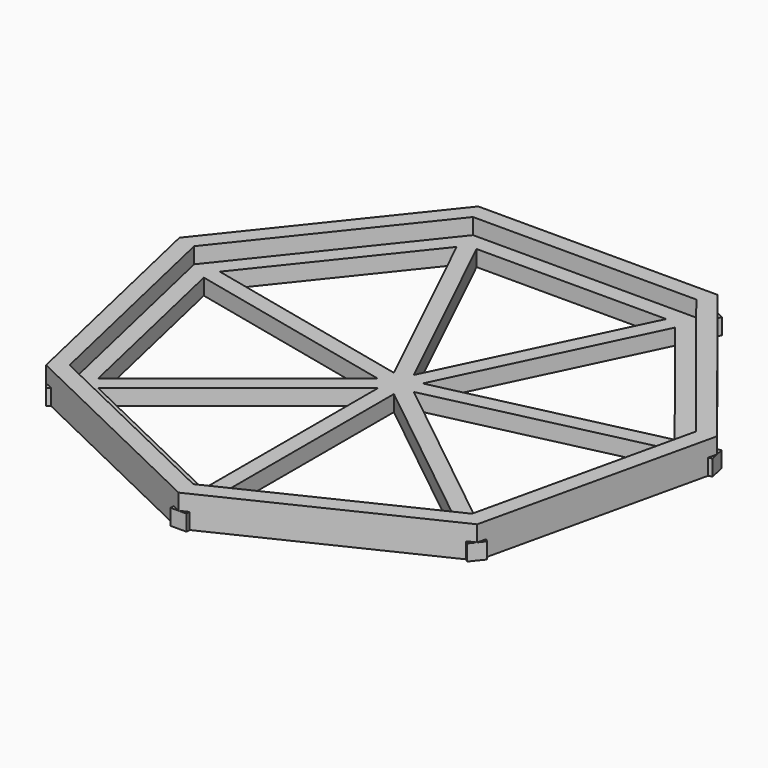
from build123d import *

# Parameters (mm, degrees)
F1_E8_W   = 109.7644269796
F1_E8_H   = 6.35
F2_DEPTH  = 3.175
F1_E7_W   = 109.7644269796
F1_E7_H   = 6.35
F3_DEPTH  = 3.175
F4_E6_W   = 109.7644269796
F4_E6_H   = 6.35
F5_DEPTH  = 3.175
F4_E5_W   = 109.7644269796
F4_E5_H   = 6.35
F6_DEPTH  = 3.175
F7_E4_W   = 109.7644269796
F7_E4_H   = 6.35
F8_DEPTH  = 3.175
F7_E3_W   = 109.7644269796
F7_E3_H   = 6.35
F9_DEPTH  = 3.175
F10_E9_W  = 109.7644269796
F10_E9_H  = 6.35
F11_DEPTH = 3.175
F12_DEPTH = 12.7
F13_DEPTH = 6.35


with BuildPart() as f2:
    # F1_E8 (on explicit) → F2 (new body, symmetric)
    with BuildSketch(Plane(origin=(0, -109.7644269796, 0), x_dir=(0, 1, 0), z_dir=(1, 0, 0))):
        with Locations((54.8822134898, 3.175)):
            Rectangle(F1_E8_W, F1_E8_H)
    extrude(amount=F2_DEPTH, both=True)

    # F1_E7 (on explicit) → F3 (join, symmetric)
    with BuildSketch(Plane(origin=(85.8172846677, -68.4370008286, 0), x_dir=(-0.7818314825, 0.6234898019, 0), z_dir=(0.6234898019, 0.7818314825, 0))):
        with Locations((54.8822134898, 3.175)):
            Rectangle(F1_E7_W, F1_E7_H)
    extrude(amount=F3_DEPTH, both=True)

    # F4_E6 (on explicit) → F5 (join, symmetric)
    with BuildSketch(Plane(origin=(107.012403627, 24.4248828067, 0), x_dir=(-0.9749279122, -0.222520934, 0), z_dir=(-0.222520934, 0.9749279122, 0))):
        with Locations((54.8822134898, 3.175)):
            Rectangle(F4_E6_W, F4_E6_H)
    extrude(amount=F5_DEPTH, both=True)

    # F4_E5 (on explicit) → F6 (join, symmetric)
    with BuildSketch(Plane(origin=(47.625, 98.8943315118, 0), x_dir=(-0.4338837391, -0.9009688679, 0), z_dir=(-0.9009688679, 0.4338837391, 0))):
        with Locations((54.8822134898, 3.175)):
            Rectangle(F4_E5_W, F4_E5_H)
    extrude(amount=F6_DEPTH, both=True)

    # F7_E4 (on explicit) → F8 (join, symmetric)
    with BuildSketch(Plane(origin=(-47.625, 98.8943315118, 0), x_dir=(0.4338837391, -0.9009688679, 0), z_dir=(-0.9009688679, -0.4338837391, 0))):
        with Locations((54.8822134898, 3.175)):
            Rectangle(F7_E4_W, F7_E4_H)
    extrude(amount=F8_DEPTH, both=True)

    # F7_E3 (on explicit) → F9 (join, symmetric)
    with BuildSketch(Plane(origin=(-107.012403627, 24.4248828067, 0), x_dir=(0.9749279122, -0.222520934, 0), z_dir=(-0.222520934, -0.9749279122, 0))):
        with Locations((54.8822134898, 3.175)):
            Rectangle(F7_E3_W, F7_E3_H)
    extrude(amount=F9_DEPTH, both=True)

    # F10_E9 (on explicit) → F11 (join, symmetric)
    with BuildSketch(Plane(origin=(-85.8172846677, -68.4370008286, 0), x_dir=(0.7818314825, 0.6234898019, 0), z_dir=(0.6234898019, -0.7818314825, 0))):
        with Locations((54.8822134898, 3.175)):
            Rectangle(F10_E9_W, F10_E9_H)
    extrude(amount=F11_DEPTH, both=True)

    # F0 (on Top) → F12 (join)
    with BuildSketch(Plane.XY):
        Polygon((44.45, 92.3013760776), (47.625, 98.8943315118), (-47.625, 98.8943315118), (-44.45, 92.3013760776), align=None)
        Polygon((99.8782433852, 22.7965572862), (107.012403627, 24.4248828067), (47.625, 98.8943315118), (44.45, 92.3013760776), align=None)
        Polygon((80.0961323565, -63.8745341067), (85.8172846677, -68.4370008286), (107.012403627, 24.4248828067), (99.8782433852, 22.7965572862), align=None)
        Polygon((0, -109.7644269796), (85.8172846677, -68.4370008286), (80.0961323565, -63.8745341067), (0, -102.4467985143), align=None)
        Polygon((-85.8172846677, -68.4370008286), (0, -109.7644269796), (0, -102.4467985143), (-80.0961323565, -63.8745341067), align=None)
        Polygon((-107.012403627, 24.4248828067), (-85.8172846677, -68.4370008286), (-80.0961323565, -63.8745341067), (-99.8782433852, 22.7965572862), align=None)
        Polygon((-47.625, 98.8943315118), (-107.012403627, 24.4248828067), (-99.8782433852, 22.7965572862), (-44.45, 92.3013760776), align=None)
    extrude(amount=F12_DEPTH)

    # F0 (on Top) → F13 (join)
    with BuildSketch(Plane.XY):
        Polygon((92.7440831434, 21.1682317658), (99.8782433852, 22.7965572862), (44.45, 92.3013760776), (41.275, 85.7084206435), align=None)
        Polygon((41.275, 85.7084206435), (44.45, 92.3013760776), (-44.45, 92.3013760776), (-41.275, 85.7084206435), align=None)
        Polygon((-44.45, 92.3013760776), (-99.8782433852, 22.7965572862), (-92.7440831434, 21.1682317658), (-41.275, 85.7084206435), align=None)
        Polygon((-99.8782433852, 22.7965572862), (-80.0961323565, -63.8745341067), (-74.3749800453, -59.3120673848), (-92.7440831434, 21.1682317658), align=None)
        Polygon((-80.0961323565, -63.8745341067), (0, -102.4467985143), (0, -95.129170049), (-74.3749800453, -59.3120673848), align=None)
        Polygon((0, -102.4467985143), (80.0961323565, -63.8745341067), (74.3749800453, -59.3120673848), (0, -95.129170049), align=None)
        Polygon((74.3749800453, -59.3120673848), (80.0961323565, -63.8745341067), (99.8782433852, 22.7965572862), (92.7440831434, 21.1682317658), align=None)
    extrude(amount=F13_DEPTH)


solid = f2.part
